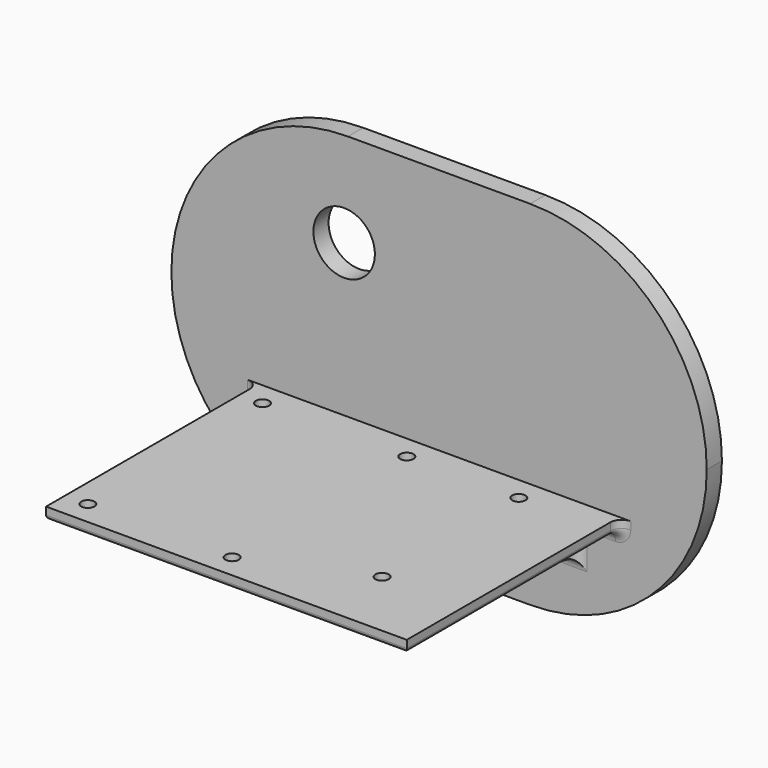
from build123d import *

# Parameters (mm, degrees)
F1_DEPTH      = 5
F2_W          = 95
F2_H          = 3
F3_DEPTH      = 70
F4_R          = 1.75
F5_DEPTH      = 25
F6_R          = 1
F8_W          = 6
F8_H          = 10
F9_DEPTH      = 50
F11_DEPTH     = 80
F12_T1_DEPTH  = 18
F12_T3_DEPTH  = 6
F12_T5_DEPTH  = 75
F12_T7_DEPTH  = 6
F12_T9_DEPTH  = 18
F12_T11_DEPTH = 2
F12_T16_DEPTH = 17.5
F12_T21_DEPTH = 17.5
F12_T26_DEPTH = 17.5
F12_T31_DEPTH = 17.5
F12_T34_ANGLE = 90
F12_T36_ANGLE = 90
F12_T41_DEPTH = 12.1485292704
F12_T45_DEPTH = 17.5
F12_T52_DEPTH = 17.5
F12_T56_DEPTH = 12.1485292704
F12_T63_DEPTH = 12.1485292704
F12_T67_DEPTH = 17.5
F12_T74_DEPTH = 17.5
F12_T78_DEPTH = 12.1485292704
F7_R          = 8.1
F13_DEPTH     = 25
F14_TEXT_SIZE = 18.0555555556
F15_DEPTH     = 1
F16_TEXT_SIZE = 13.8888888889
F17_DEPTH     = 1


# Not quite as in the source:
# - a fillet or chamfer that OpenCascade refuses, or shapes differently, is made with other operations: its cross-section is extruded or revolved along the edge and cut away or added
# - Text() gives the source's letters only with a copy of the font that has no kerning and outlines rounded to 1/6400 em; it was checked with that copy


with BuildPart() as f1:
    # F0 (on Front) → F1 (new body)
    with BuildSketch(Plane.XZ):
        with BuildLine():
            ThreePointArc((70.5, 0), (56.8804653252, 32.8804653252), (24, 46.5))
            Line((24, 46.5), (-24, 46.5))
            ThreePointArc((-24, 46.5), (-56.8804653252, 32.8804653252), (-70.5, 0))
            ThreePointArc((-70.5, 0), (-56.8804653252, -32.8804653252), (-24, -46.5))
            Line((-24, -46.5), (24, -46.5))
            ThreePointArc((24, -46.5), (56.8804653252, -32.8804653252), (70.5, 0))
        make_face()
    extrude(amount=F1_DEPTH)

    # F2 (on face) → F3 (join)
    with BuildSketch(Plane.XZ.offset(5)):
        with Locations((0, -20)):
            Rectangle(F2_W, F2_H)
    extrude(amount=F3_DEPTH)

    # F4 (on face) → F5 (cut)
    with BuildSketch(Plane.XY.offset(-18.5)):
        with Locations((-3.5, -68.75)):
            Circle(F4_R)
        with Locations((-41.5, -68.75)):
            Circle(F4_R)
        with Locations((-41.5, -11.25)):
            Circle(F4_R)
        with Locations((-3.5, -11.25)):
            Circle(F4_R)
        with Locations((26, -56.25)):
            Circle(F4_R)
        with Locations((26, -11.25)):
            Circle(F4_R)
    extrude(amount=-F5_DEPTH, mode=Mode.SUBTRACT)

    # F6
    f6_edges = [f1.edges().sort_by_distance(p)[0] for p in [
        (47.5, -40, -21.5),
        (-47.5, -40, -21.5),
        (0, -75, -21.5),
    ]]
    fillet(f6_edges, radius=F6_R)

    # F8 (on face) → F9 (join)
    with BuildSketch(Plane.XZ.offset(5)):
        with Locations((-33, -26.5)):
            Rectangle(F8_W, F8_H)
        with Locations((33, -26.5)):
            Rectangle(F8_W, F8_H)
    extrude(amount=F9_DEPTH)

    # F10 (on face) → F11 (cut)
    with BuildSketch(Plane(origin=(-36, 0, 0), x_dir=(0, -1, 0), z_dir=(-1, 0, 0))):
        Polygon((55, -31.5), (55, -21.5), (5, -31.5), align=None)
    extrude(amount=-F11_DEPTH, mode=Mode.SUBTRACT)

    # F12: fillet of radius 3 on 9 edges, made by hand

    # F12_s2 → F12_t1 (join)
    with BuildSketch(Plane.YZ.offset(-46.5)):
        with BuildLine():
            ThreePointArc((-5, -24.5), (-5.8786796564, -22.3786796564), (-8, -21.5))
            Line((-8, -21.5), (-5, -21.5))
            Line((-5, -21.5), (-5, -24.5))
        make_face()
    extrude(amount=F12_T1_DEPTH)

    # F12_s4 → F12_t3 (join)
    with BuildSketch(Plane.YZ.offset(-36)):
        with BuildLine():
            ThreePointArc((-5, -33.9594117082), (-5.679973576, -32.0574449913), (-7.4116515946, -31.0176696811))
            Line((-7.4116515946, -31.0176696811), (-5, -31.5))
            Line((-5, -31.5), (-5, -33.9594117082))
        make_face()
    extrude(amount=F12_T3_DEPTH)

    # F12_s6 → F12_t5 (join)
    with BuildSketch(Plane.YZ.offset(-37.5)):
        with BuildLine():
            ThreePointArc((-5, -24.5), (-5.8786796564, -22.3786796564), (-8, -21.5))
            Line((-8, -21.5), (-5, -21.5))
            Line((-5, -21.5), (-5, -24.5))
        make_face()
    extrude(amount=F12_T5_DEPTH)

    # F12_s8 → F12_t7 (join)
    with BuildSketch(Plane.YZ.offset(30)):
        with BuildLine():
            ThreePointArc((-5, -33.9594117082), (-5.679973576, -32.0574449913), (-7.4116515946, -31.0176696811))
            Line((-7.4116515946, -31.0176696811), (-5, -31.5))
            Line((-5, -31.5), (-5, -33.9594117082))
        make_face()
    extrude(amount=F12_T7_DEPTH)

    # F12_s10 → F12_t9 (join)
    with BuildSketch(Plane.YZ.offset(28.5)):
        with BuildLine():
            ThreePointArc((-5, -24.5), (-5.8786796564, -22.3786796564), (-8, -21.5))
            Line((-8, -21.5), (-5, -21.5))
            Line((-5, -21.5), (-5, -24.5))
        make_face()
    extrude(amount=F12_T9_DEPTH)

    # F12_s12 → F12_t11 (join)
    with BuildSketch(Plane.XY.offset(-20.5)):
        with BuildLine():
            ThreePointArc((50.5, -5), (48.3786796564, -5.8786796564), (47.5, -8))
            Line((47.5, -8), (47.5, -5))
            Line((47.5, -5), (50.5, -5))
        make_face()
        with BuildLine():
            ThreePointArc((-50.5, -5), (-48.3786796564, -5.8786796564), (-47.5, -8))
            Line((-47.5, -8), (-47.5, -5))
            Line((-47.5, -5), (-50.5, -5))
        make_face()
    extrude(amount=F12_T11_DEPTH)


with BuildPart() as f12_tool14:
    # F12_s15 → F12_t16 (new body)
    with BuildSketch(Plane.XY.offset(-21.5)):
        with BuildLine():
            ThreePointArc((-39, -5), (-36.8786796564, -5.8786796564), (-36, -8))
            Line((-36, -8), (-36, -5))
            Line((-36, -5), (-39, -5))
        make_face()
    extrude(amount=-F12_T16_DEPTH)

    split(bisect_by=Plane(origin=(0, -6.25, -31.25), x_dir=(1, 0, 0), z_dir=(0, 0.1961161351, 0.9805806757)), keep=Keep.TOP)


with BuildPart() as f1_1:
    add(f1.part)

    # F12_t13: union F12_tool14
    add(f12_tool14.part)


with BuildPart() as f12_tool19:
    # F12_s20 → F12_t21 (new body)
    with BuildSketch(Plane.XY.offset(-39)):
        with BuildLine():
            ThreePointArc((-27, -5), (-29.1213203436, -5.8786796564), (-30, -8))
            Line((-30, -8), (-30, -5))
            Line((-30, -5), (-27, -5))
        make_face()
    extrude(amount=F12_T21_DEPTH)

    split(bisect_by=Plane(origin=(0, -6.25, -31.25), x_dir=(1, 0, 0), z_dir=(0, 0.1961161351, 0.9805806757)), keep=Keep.TOP)


with BuildPart() as f1_2:
    add(f1_1.part)

    # F12_t18: union F12_tool19
    add(f12_tool19.part)


with BuildPart() as f12_tool24:
    # F12_s25 → F12_t26 (new body)
    with BuildSketch(Plane.XY.offset(-21.5)):
        with BuildLine():
            ThreePointArc((27, -5), (29.1213203436, -5.8786796564), (30, -8))
            Line((30, -8), (30, -5))
            Line((30, -5), (27, -5))
        make_face()
    extrude(amount=-F12_T26_DEPTH)

    split(bisect_by=Plane(origin=(0, -6.25, -31.25), x_dir=(1, 0, 0), z_dir=(0, 0.1961161351, 0.9805806757)), keep=Keep.TOP)


with BuildPart() as f1_3:
    add(f1_2.part)

    # F12_t23: union F12_tool24
    add(f12_tool24.part)


with BuildPart() as f12_tool29:
    # F12_s30 → F12_t31 (new body)
    with BuildSketch(Plane.XY.offset(-39)):
        with BuildLine():
            ThreePointArc((39, -5), (36.8786796564, -5.8786796564), (36, -8))
            Line((36, -8), (36, -5))
            Line((36, -5), (39, -5))
        make_face()
    extrude(amount=F12_T31_DEPTH)

    split(bisect_by=Plane(origin=(0, -6.25, -31.25), x_dir=(1, 0, 0), z_dir=(0, 0.1961161351, 0.9805806757)), keep=Keep.TOP)


with BuildPart() as f1_4:
    add(f1_3.part)

    # F12_t28: union F12_tool29
    add(f12_tool29.part)

    # F12_s33 → F12_t34 (revolve)
    with BuildSketch(Plane.XY.offset(-20.5)):
        with BuildLine():
            ThreePointArc((50.5, -5), (48.3786796564, -5.8786796564), (47.5, -8))
            Line((47.5, -8), (47.5, -5))
            Line((47.5, -5), (50.5, -5))
        make_face()
    revolve(axis=Axis((46.5, -5, -20.5), (0, 1, 0)), revolution_arc=F12_T34_ANGLE)

    # F12_s35 → F12_t36 (revolve)
    with BuildSketch(Plane.XY.offset(-20.5)):
        with BuildLine():
            ThreePointArc((-50.5, -5), (-48.3786796564, -5.8786796564), (-47.5, -8))
            Line((-47.5, -8), (-47.5, -5))
            Line((-47.5, -5), (-50.5, -5))
        make_face()
    revolve(axis=Axis((-46.5, -5, -20.5), (0, -1, 0)), revolution_arc=F12_T36_ANGLE)


with BuildPart() as f12_tool39:
    # F12_s40 → F12_t41 (new body)
    with BuildSketch(Plane.YZ.offset(-42.1485292704)):
        with BuildLine():
            ThreePointArc((-5, -33.9594117082), (-5.679973576, -32.0574449913), (-7.4116515946, -31.0176696811))
            Line((-7.4116515946, -31.0176696811), (-5, -31.5))
            Line((-5, -31.5), (-5, -33.9594117082))
        make_face()
    extrude(amount=F12_T41_DEPTH)

    split(bisect_by=Plane.YZ.offset(-36), keep=Keep.BOTTOM)


with BuildPart() as f12_tool43:
    # F12_s44 → F12_t45 (new body)
    with BuildSketch(Plane.XY.offset(-21.5)):
        with BuildLine():
            ThreePointArc((-39, -5), (-36.8786796564, -5.8786796564), (-36, -8))
            Line((-36, -8), (-36, -5))
            Line((-36, -5), (-39, -5))
        make_face()
    extrude(amount=-F12_T45_DEPTH)

    split(bisect_by=Plane(origin=(0, -6.25, -31.25), x_dir=(1, 0, 0), z_dir=(0, -0.1961161351, -0.9805806757)), keep=Keep.TOP)


with BuildPart() as f12_tool39_1:
    add(f12_tool39.part)

    # F12_t47: intersect F12_tool43
    add(f12_tool43.part, mode=Mode.INTERSECT)


with BuildPart() as f1_5:
    add(f1_4.part)

    # F12_t37: union F12_tool39
    add(f12_tool39_1.part)


with BuildPart() as f12_tool50:
    # F12_s51 → F12_t52 (new body)
    with BuildSketch(Plane.XY.offset(-39)):
        with BuildLine():
            ThreePointArc((-27, -5), (-29.1213203436, -5.8786796564), (-30, -8))
            Line((-30, -8), (-30, -5))
            Line((-30, -5), (-27, -5))
        make_face()
    extrude(amount=F12_T52_DEPTH)

    split(bisect_by=Plane(origin=(0, -6.25, -31.25), x_dir=(1, 0, 0), z_dir=(0, -0.1961161351, -0.9805806757)), keep=Keep.TOP)


with BuildPart() as f12_tool54:
    # F12_s55 → F12_t56 (new body)
    with BuildSketch(Plane.YZ.offset(-36)):
        with BuildLine():
            ThreePointArc((-5, -33.9594117082), (-5.679973576, -32.0574449913), (-7.4116515946, -31.0176696811))
            Line((-7.4116515946, -31.0176696811), (-5, -31.5))
            Line((-5, -31.5), (-5, -33.9594117082))
        make_face()
    extrude(amount=F12_T56_DEPTH)

    split(bisect_by=Plane.YZ.offset(-30), keep=Keep.TOP)


with BuildPart() as f12_tool50_1:
    add(f12_tool50.part)

    # F12_t58: intersect F12_tool54
    add(f12_tool54.part, mode=Mode.INTERSECT)


with BuildPart() as f1_6:
    add(f1_5.part)

    # F12_t48: union F12_tool50
    add(f12_tool50_1.part)


with BuildPart() as f12_tool61:
    # F12_s62 → F12_t63 (new body)
    with BuildSketch(Plane.YZ.offset(23.8514707296)):
        with BuildLine():
            ThreePointArc((-5, -33.9594117082), (-5.679973576, -32.0574449913), (-7.4116515946, -31.0176696811))
            Line((-7.4116515946, -31.0176696811), (-5, -31.5))
            Line((-5, -31.5), (-5, -33.9594117082))
        make_face()
    extrude(amount=F12_T63_DEPTH)

    split(bisect_by=Plane.YZ.offset(30), keep=Keep.BOTTOM)


with BuildPart() as f12_tool65:
    # F12_s66 → F12_t67 (new body)
    with BuildSketch(Plane.XY.offset(-21.5)):
        with BuildLine():
            ThreePointArc((27, -5), (29.1213203436, -5.8786796564), (30, -8))
            Line((30, -8), (30, -5))
            Line((30, -5), (27, -5))
        make_face()
    extrude(amount=-F12_T67_DEPTH)

    split(bisect_by=Plane(origin=(0, -6.25, -31.25), x_dir=(1, 0, 0), z_dir=(0, -0.1961161351, -0.9805806757)), keep=Keep.TOP)


with BuildPart() as f12_tool61_1:
    add(f12_tool61.part)

    # F12_t69: intersect F12_tool65
    add(f12_tool65.part, mode=Mode.INTERSECT)


with BuildPart() as f1_7:
    add(f1_6.part)

    # F12_t59: union F12_tool61
    add(f12_tool61_1.part)


with BuildPart() as f12_tool72:
    # F12_s73 → F12_t74 (new body)
    with BuildSketch(Plane.XY.offset(-39)):
        with BuildLine():
            ThreePointArc((39, -5), (36.8786796564, -5.8786796564), (36, -8))
            Line((36, -8), (36, -5))
            Line((36, -5), (39, -5))
        make_face()
    extrude(amount=F12_T74_DEPTH)

    split(bisect_by=Plane(origin=(0, -6.25, -31.25), x_dir=(1, 0, 0), z_dir=(0, -0.1961161351, -0.9805806757)), keep=Keep.TOP)


with BuildPart() as f12_tool76:
    # F12_s77 → F12_t78 (new body)
    with BuildSketch(Plane.YZ.offset(30)):
        with BuildLine():
            ThreePointArc((-5, -33.9594117082), (-5.679973576, -32.0574449913), (-7.4116515946, -31.0176696811))
            Line((-7.4116515946, -31.0176696811), (-5, -31.5))
            Line((-5, -31.5), (-5, -33.9594117082))
        make_face()
    extrude(amount=F12_T78_DEPTH)

    split(bisect_by=Plane.YZ.offset(36), keep=Keep.TOP)


with BuildPart() as f12_tool72_1:
    add(f12_tool72.part)

    # F12_t80: intersect F12_tool76
    add(f12_tool76.part, mode=Mode.INTERSECT)


with BuildPart() as f1_8:
    add(f1_7.part)

    # F12_t70: union F12_tool72
    add(f12_tool72_1.part)

    # F7 (on face) → F13 (cut)
    with BuildSketch(Plane.XZ.offset(5)):
        with Locations((-25, 21.5)):
            Circle(F7_R)
    extrude(amount=-F13_DEPTH, mode=Mode.SUBTRACT)

    # F14 (on face) → F15 (cut)
    with BuildSketch(Plane(origin=(0, 0, 0), x_dir=(-1, 0, 0), z_dir=(0, 1, 0))):
        with Locations((-61.4100477431, -16.5)):
            Text('Omri Forkosh', F14_TEXT_SIZE, font='Open Sans', font_style=FontStyle.BOLD, text_align=(TextAlign.LEFT, TextAlign.BOTTOM))
    extrude(amount=-F15_DEPTH, mode=Mode.SUBTRACT)

    # F16 (on face) → F17 (cut)
    with BuildSketch(Plane(origin=(0, 0, 0), x_dir=(-1, 0, 0), z_dir=(0, 1, 0))):
        with Locations((-31.005859375, -31.5)):
            Text('Auto Bath', F16_TEXT_SIZE, font='Tinos', font_style=FontStyle.BOLD, text_align=(TextAlign.LEFT, TextAlign.BOTTOM))
    extrude(amount=-F17_DEPTH, mode=Mode.SUBTRACT)


solid = f1_8.part
